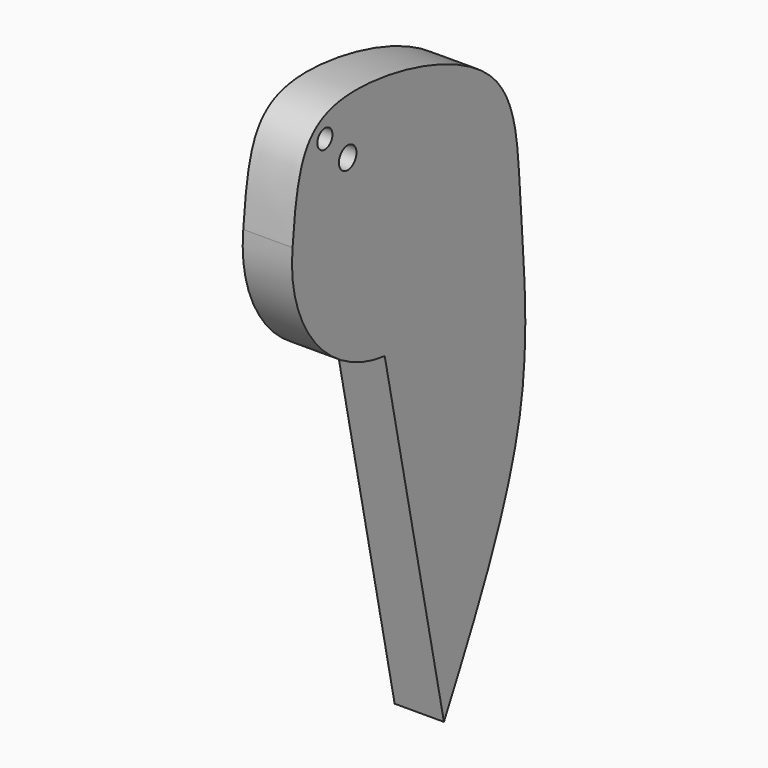
from build123d import *

# Parameters (mm, degrees)
F1_DEPTH = 12.7
F2_R     = 2.4323517369
F3_DEPTH = 25.4
F4_R     = 2.8332069334
F5_DEPTH = 25.4


# Not quite as in the source:
# - a length typed as a fraction of an inch, garbled in the dataset ("3 / 203.2 mm" for 3/8 in), is restored


with BuildPart() as f1:
    # F0 (on Right) → F1 (new body)
    with BuildSketch(Plane.YZ):
        with BuildLine():
            ThreePointArc((-73.3486190438, 75.1153677702), (-66.1138740034, 50.6307129788), (-43.6681210995, 38.4640358388))
            Line((-43.6681210995, 38.4640358388), (-24.5922897011, -52.2894561291))
            add(Edge.make_bspline(
                [(-73.3486190438, 75.1153677702), (-72.6117781214, 83.1247650404), (-71.2247390094, 98.2017605478), (-52.9853467307, 105.9270950428), (-1.0990052853, 92.7895590782), (-0.6789523299, 55.3079359595), (5.4837017479, 5.8690932712), (-14.0842244334, -31.9697990361), (-24.5922897011, -52.2894561291)],
                knots=[0, 0, 0, 0, 0.127846329, 0.2406596231, 0.4286554949, 0.58558405, 0.7774567519, 1, 1, 1, 1], degree=3))
        make_face()
    extrude(amount=F1_DEPTH)

    # F2 (on face) → F3 (cut)
    with BuildSketch(Plane.YZ.offset(12.7)):
        with Locations((-62.9347339272, 95.5596640706)):
            Circle(F2_R)
    extrude(amount=-F3_DEPTH, mode=Mode.SUBTRACT)

    # F4 (on face) → F5 (cut)
    with BuildSketch(Plane.YZ.offset(12.7)):
        with Locations((-55.5986575782, 88.2956758142)):
            Circle(F4_R)
    extrude(amount=-F5_DEPTH, mode=Mode.SUBTRACT)


solid = f1.part
